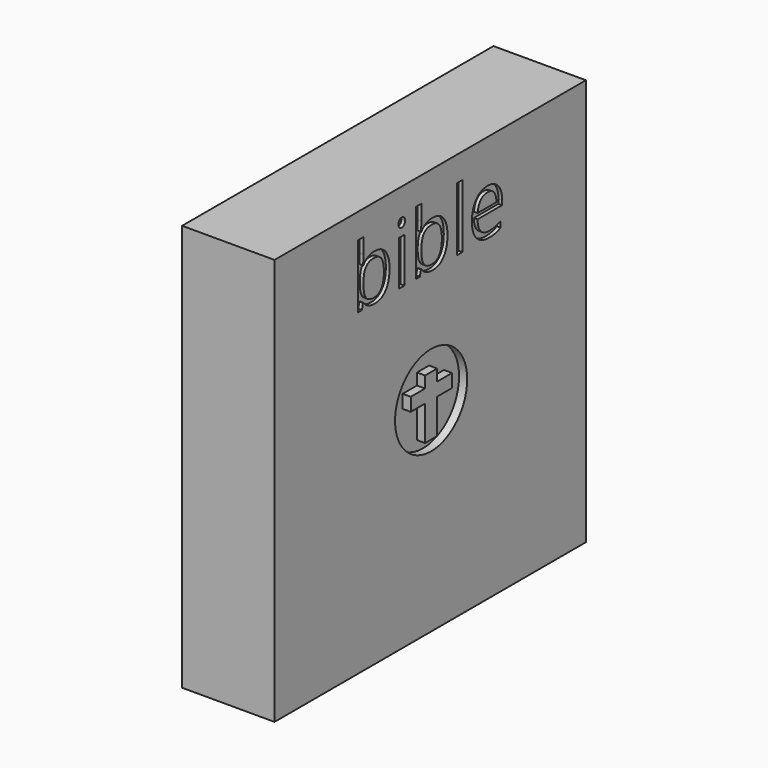
from build123d import *

# Parameters (mm, degrees)
F0_W         = 105.2752286196
F0_H         = 110.0229360163
F1_DEPTH     = 12.5
F3_R         = 12.20057076
F4_DEPTH     = 27.2
F5_TEXT_SIZE = 22.6293121361
F6_DEPTH     = 26


# Not quite as in the source:
# - Text() gives the source's letters only with a copy of the font that has no kerning and outlines rounded to 1/6400 em; it was checked with that copy


with BuildPart() as f1:
    # F0 (on Right) → F1 (new body, symmetric)
    with BuildSketch(Plane.YZ):
        with Locations((-0.3096349537, -0.1032110304)):
            Rectangle(F0_W, F0_H)
    extrude(amount=F1_DEPTH, both=True)

    # F3 (on offset) → F4 (cut)
    with BuildSketch(Plane.YZ.offset(37.5)):
        Circle(F3_R)
        Polygon((-2.0366383251, 3.5883623641), (-2.0366383251, 6.691810675), (2.0366383251, 6.691810675), (2.0366383251, 3.5883623641), (7.0797409862, 3.5883623641), (7.0797409862, 0), (2.0366383251, 0), (2.0366383251, -9.4073284417), (-2.0366383251, -9.4073284417), (-2.0366383251, 0), (-6.8857762963, 0), (-6.8857762963, 3.5883623641), align=None, mode=Mode.SUBTRACT)
    extrude(amount=-F4_DEPTH, mode=Mode.SUBTRACT)

    # F5 (on offset) → F6 (cut)
    with BuildSketch(Plane.YZ.offset(37.5)):
        with Locations((-26.6702575609, 30.937500298)):
            Text('bible', F5_TEXT_SIZE, font='Open Sans', text_align=(TextAlign.LEFT, TextAlign.BOTTOM))
    extrude(amount=-F6_DEPTH, mode=Mode.SUBTRACT)


solid = f1.part
